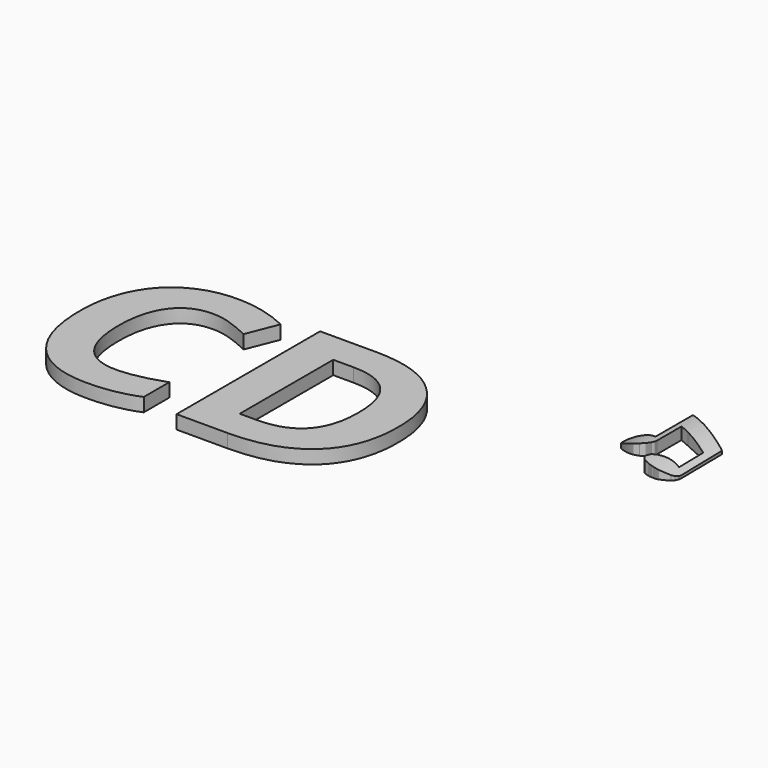
from build123d import *

# Parameters (mm, degrees)
F0_TEXT_SIZE = 55.5555555556
F1_DEPTH     = 3
F3_DEPTH     = 3
F4_R         = 20.7673128918
F4_R_2       = 15.7673128918
F5_DEPTH     = 57.7


# Not quite as in the source:
# - ends of sketch curves that miss each other by under 0.0002 mm in the source are joined
# - Text() gives the source's letters only with a copy of the font that has no kerning and outlines rounded to 1/6400 em; it was checked with that copy


with BuildPart() as f1:
    # F0 (on Top) → F1 (new body)
    with BuildSketch(Plane.XY):
        with Locations((-80.4245307969, -3.7874889469)):
            Text('CD', F0_TEXT_SIZE, font='Open Sans', font_style=FontStyle.BOLD, text_align=(TextAlign.LEFT, TextAlign.BOTTOM))
    extrude(amount=F1_DEPTH)


with BuildPart() as f3:
    # F2 (on Top) → F3 (new body)
    with BuildSketch(Plane.XY):
        with BuildLine():
            Line((39.3247738246, 36.0116689029), (39.3743909621, 36.2647128176))
            Line((39.3743909621, 36.2647128176), (39.230365836, 47.7867220706))
            Line((39.230365836, 47.7867220706), (38.7548213133, 48.0584619469))
            Line((38.7548213133, 48.0584619469), (34.7778010762, 49.8260265663))
            Line((34.7778010762, 49.8260265663), (29.5487559961, 52.1827793226))
            Line((29.5487559961, 52.1827793226), (29.5038227655, 52.2030660924))
            Line((29.5038227655, 52.2030660924), (29.4585028976, 52.2194459878))
            Line((29.4585028976, 52.2194459878), (29.4128327178, 52.2322895712))
            Line((29.4128327178, 52.2322895712), (29.3668489693, 52.2419671958))
            Line((29.3668489693, 52.2419671958), (29.2740879473, 52.2533066095))
            ThreePointArc((29.2740879473, 52.2533066095), (29.2272522118, 52.2342629258), (29.1805133583, 52.2149826878))
            Line((29.1805133583, 52.2149826878), (29.1805133583, 42.019283022))
            Line((29.1805133583, 42.019283022), (28.2967309443, 42.2402287299))
            Line((28.2967309443, 42.2402287299), (28.1722063697, 42.2519633404))
            Line((28.1722063697, 42.2519633404), (28.0475872234, 42.2598334564))
            Line((28.0475872234, 42.2598334564), (27.922900854, 42.2640691395))
            Line((27.922900854, 42.2640691395), (27.7981741925, 42.264900034))
            Line((27.7981741925, 42.264900034), (27.5487093873, 42.2572664516))
            Line((27.5487093873, 42.2572664516), (27.2994103435, 42.2387706979))
            Line((27.2994103435, 42.2387706979), (27.050494388, 42.2112511793))
            Line((27.050494388, 42.2112511793), (26.8021792652, 42.1765460932))
            Line((26.8021792652, 42.1765460932), (26.5546823021, 42.1364934284))
            Line((26.5546823021, 42.1364934284), (26.3082208257, 42.0929315913))
            Line((26.3082208257, 42.0929315913), (25.9267655038, 41.970998656))
            Line((25.9267655038, 41.970998656), (25.7359616427, 41.9096623568))
            Line((25.7359616427, 41.9096623568), (25.5469093406, 41.8448949643))
            Line((25.5469093406, 41.8448949643), (25.3609601582, 41.7743077612))
            Line((25.3609601582, 41.7743077612), (25.1794662823, 41.6955124475))
            Line((25.1794662823, 41.6955124475), (25.0908123426, 41.6522902751))
            Line((25.0908123426, 41.6522902751), (25.0037790647, 41.6061205148))
            Line((25.0037790647, 41.6061205148), (24.9185353415, 41.5567044204))
            Line((24.9185353415, 41.5567044204), (24.8352504835, 41.5037434544))
            Line((24.8352504835, 41.5037434544), (24.6401272235, 41.3687383355))
            Line((24.6401272235, 41.3687383355), (24.45143087, 41.2265528683))
            Line((24.45143087, 41.2265528683), (24.3599182774, 41.152291984))
            Line((24.3599182774, 41.152291984), (24.2705230044, 41.0756655556))
            Line((24.2705230044, 41.0756655556), (24.1834151965, 40.9964833958))
            Line((24.1834151965, 40.9964833958), (24.098765208, 40.9145553175))
            Line((24.098765208, 40.9145553175), (24.0522403343, 40.8649484097))
            Line((24.0522403343, 40.8649484097), (24.0093336095, 40.8132417186))
            Line((24.0093336095, 40.8132417186), (23.969621862, 40.7596809637))
            Line((23.969621862, 40.7596809637), (23.9326817114, 40.7045118643))
            Line((23.9326817114, 40.7045118643), (23.8654230967, 40.5903308826))
            Line((23.8654230967, 40.5903308826), (23.8041711396, 40.4726641105))
            Line((23.8041711396, 40.4726641105), (23.7747783504, 40.4083789708))
            Line((23.7747783504, 40.4083789708), (23.750076775, 40.3429462364))
            Line((23.750076775, 40.3429462364), (23.729769546, 40.2764753014))
            Line((23.729769546, 40.2764753014), (23.7135591698, 40.2090766037))
            Line((23.7135591698, 40.2090766037), (23.7011491965, 40.1408597464))
            Line((23.7011491965, 40.1408597464), (23.6922425501, 40.0719349585))
            Line((23.6922425501, 40.0719349585), (23.6837509334, 39.9324010469))
            Line((23.6837509334, 39.9324010469), (23.6857089635, 39.791354615))
            Line((23.6857089635, 39.791354615), (23.6957406578, 39.6496752002))
            Line((23.6957406578, 39.6496752002), (23.7114704513, 39.5082425485))
            Line((23.7114704513, 39.5082425485), (23.7305225703, 39.3679361973))
            Line((23.7305225703, 39.3679361973), (24.0251166387, 38.8523966297))
            Line((24.0251166387, 38.8523966297), (24.3933592765, 38.5578025613))
            Line((24.3933592765, 38.5578025613), (24.5665423283, 38.490692589))
            Line((24.5665423283, 38.490692589), (24.7411316378, 38.4275066101))
            Line((24.7411316378, 38.4275066101), (24.9170069549, 38.3685316797))
            Line((24.9170069549, 38.3685316797), (25.0940478208, 38.3140556882))
            Line((25.0940478208, 38.3140556882), (25.2721339853, 38.2643658996))
            Line((25.2721339853, 38.2643658996), (25.4511451985, 38.2197502044))
            Line((25.4511451985, 38.2197502044), (25.6309607928, 38.1804958664))
            Line((25.6309607928, 38.1804958664), (25.8114607268, 38.1468903586))
            Line((25.8114607268, 38.1468903586), (25.9925245418, 38.1192213624))
            Line((25.9925245418, 38.1192213624), (26.1740319876, 38.0977761419))
            Line((26.1740319876, 38.0977761419), (26.3558626054, 38.0828427963))
            Line((26.3558626054, 38.0828427963), (26.5378961452, 38.0747081719))
            Line((26.5378961452, 38.0747081719), (26.7200121482, 38.073660368))
            Line((26.7200121482, 38.073660368), (26.9020901555, 38.0799864398))
            Line((26.9020901555, 38.0799864398), (27.0840101258, 38.0939742776))
            Line((27.0840101258, 38.0939742776), (27.2656516003, 38.1159113542))
            Line((27.2656516003, 38.1159113542), (28.4440280829, 38.484153992))
            Line((28.4440280829, 38.484153992), (29.4014588575, 39.0733421288))
            Line((29.4014588575, 39.0733421288), (29.4928545403, 39.14855207))
            Line((29.4928545403, 39.14855207), (29.5817873934, 39.2259663869))
            Line((29.5817873934, 39.2259663869), (29.6682686901, 39.3055748498))
            Line((29.6682686901, 39.3055748498), (29.7523099127, 39.387367438))
            Line((29.7523099127, 39.387367438), (29.833921917, 39.4713341306))
            Line((29.833921917, 39.4713341306), (29.9131159765, 39.5574651154))
            Line((29.9131159765, 39.5574651154), (29.9899035734, 39.6457499543))
            Line((29.9899035734, 39.6457499543), (30.0642955637, 39.736178835))
            Line((30.0642955637, 39.736178835), (30.3588896321, 40.3253669719))
            Line((30.3588896321, 40.3253669719), (30.4142879582, 40.6008596522))
            Line((30.4142879582, 40.6008596522), (30.46095375, 40.87729283))
            Line((30.46095375, 40.87729283), (30.46095375, 47.5719176752))
            Line((30.46095375, 47.5719176752), (32.7156423884, 46.585491396))
            Line((32.7156423884, 46.585491396), (37.9446874685, 44.2287388485))
            Line((37.9446874685, 44.2287388485), (38.0183360378, 37.453074648))
            Line((38.0183360378, 37.453074648), (37.5027964703, 37.6003717866))
            Line((37.5027964703, 37.6003717866), (37.3299910788, 37.630983569))
            Line((37.3299910788, 37.630983569), (37.1561278625, 37.6546408896))
            Line((37.1561278625, 37.6546408896), (36.9814341693, 37.6717625358))
            Line((36.9814341693, 37.6717625358), (36.8061375556, 37.6827681303))
            Line((36.8061375556, 37.6827681303), (36.6304657868, 37.6880775045))
            Line((36.6304657868, 37.6880775045), (36.4546464194, 37.6881094459))
            Line((36.4546464194, 37.6881094459), (36.2789065924, 37.6832839947))
            Line((36.2789065924, 37.6832839947), (36.1034744886, 37.6740201472))
            Line((36.1034744886, 37.6740201472), (35.9276567913, 37.6591630016))
            Line((35.9276567913, 37.6591630016), (35.7528866892, 37.6376096396))
            Line((35.7528866892, 37.6376096396), (35.5792284826, 37.6096412709))
            Line((35.5792284826, 37.6096412709), (35.4067466807, 37.5755391053))
            Line((35.4067466807, 37.5755391053), (35.2355055838, 37.5355845612))
            Line((35.2355055838, 37.5355845612), (35.0655692836, 37.490058431))
            Line((35.0655692836, 37.490058431), (34.8970022892, 37.439242342))
            Line((34.8970022892, 37.439242342), (34.729868901, 37.3834170864))
            Line((34.729868901, 37.3834170864), (34.5642332106, 37.3228642915))
            Line((34.5642332106, 37.3228642915), (34.4001599359, 37.2578649583))
            Line((34.4001599359, 37.2578649583), (34.2377129598, 37.1887000879))
            Line((34.2377129598, 37.1887000879), (34.0769570002, 37.1156510988))
            Line((34.0769570002, 37.1156510988), (33.9179561486, 37.0389992007))
            Line((33.9179561486, 37.0389992007), (33.7607747056, 36.9590256035))
            Line((33.7607747056, 36.9590256035), (33.6054771801, 36.8760115168))
            Line((33.6054771801, 36.8760115168), (33.4521276639, 36.7902379418))
            Line((33.4521276639, 36.7902379418), (32.7892909577, 36.201049805))
            Line((32.7892909577, 36.201049805), (32.4946968892, 35.4645645295))
            Line((32.4946968892, 35.4645645295), (32.4852161323, 35.3716786644))
            Line((32.4852161323, 35.3716786644), (32.4805695948, 35.2781861211))
            Line((32.4805695948, 35.2781861211), (32.4810094678, 35.1845081923))
            Line((32.4810094678, 35.1845081923), (32.4867885689, 35.0910661708))
            Line((32.4867885689, 35.0910661708), (32.4981592977, 34.9982809317))
            Line((32.4981592977, 34.9982809317), (32.5153738454, 34.9065739765))
            Line((32.5153738454, 34.9065739765), (32.5386850295, 34.8163663893))
            Line((32.5386850295, 34.8163663893), (32.5683452498, 34.728079254))
            Line((32.5683452498, 34.728079254), (33.0102364568, 34.1388911171))
            Line((33.0102364568, 34.1388911171), (33.5257762332, 33.8442970487))
            Line((33.5257762332, 33.8442970487), (34.4832070078, 33.5497029802))
            Line((34.4832070078, 33.5497029802), (34.7428805421, 33.5274767607))
            Line((34.7428805421, 33.5274767607), (35.0031822577, 33.5094972889))
            Line((35.0031822577, 33.5094972889), (35.2635259356, 33.4981313618))
            Line((35.2635259356, 33.4981313618), (35.5233255655, 33.4957459847))
            Line((35.5233255655, 33.4957459847), (35.6528384299, 33.498660796))
            Line((35.6528384299, 33.498660796), (35.7819953458, 33.504708372))
            Line((35.7819953458, 33.504708372), (35.9107234533, 33.5141845361))
            Line((35.9107234533, 33.5141845361), (36.0389492664, 33.5273853205))
            Line((36.0389492664, 33.5273853205), (36.1665997162, 33.5446065488))
            Line((36.1665997162, 33.5446065488), (36.2936013168, 33.5661440445))
            Line((36.2936013168, 33.5661440445), (36.4198809995, 33.5922936311))
            Line((36.4198809995, 33.5922936311), (36.5453654869, 33.6233515495))
            ThreePointArc((36.5453654869, 33.6233515495), (37.5450050942, 34.0640490429), (38.4906063256, 34.6111614048))
            Line((38.4906063256, 34.6111614048), (38.9757668125, 35.0963218917))
            Line((38.9757668125, 35.0963218917), (39.2703608809, 35.7591585979))
            Line((39.2703608809, 35.7591585979), (39.3247738246, 36.0116689029))
        make_face()
    extrude(amount=F3_DEPTH)

    # F4 (on Front) → F5 (cut)
    with BuildSketch(Plane.XZ):
        with Locations((31.5360359177, -13.0694905352)):
            Circle(F4_R)
        with Locations((31.5360359177, -13.0694905352)):
            Circle(F4_R_2, mode=Mode.SUBTRACT)
    extrude(amount=-F5_DEPTH, mode=Mode.SUBTRACT)


solid = Compound([f1.part, f3.part])
